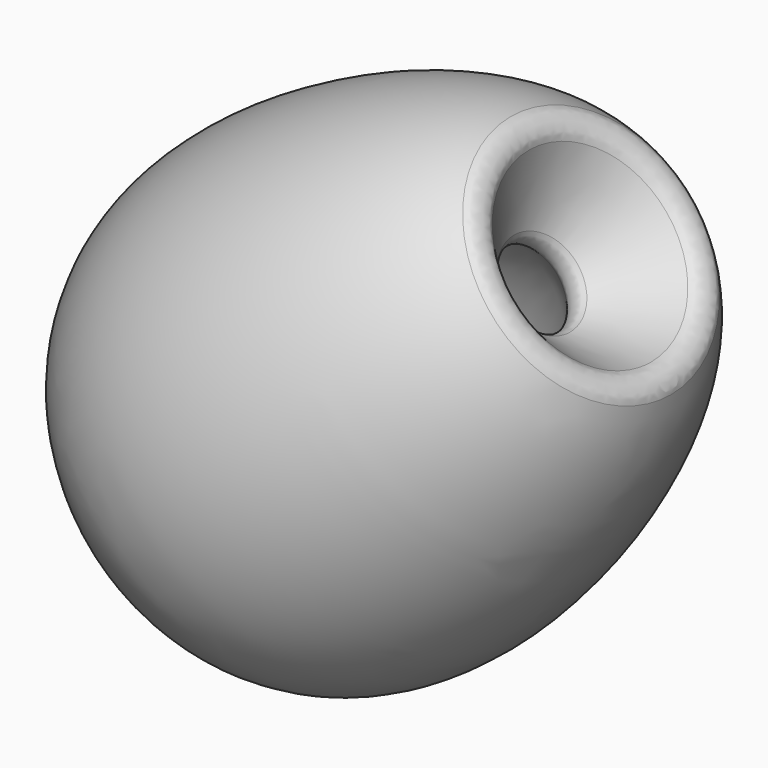
from build123d import *

# Parameters (mm, degrees)
F2_R = 12.7


# Not quite as in the source:
# - the dataset's text gives a spline's control points without its knots; the knots are read off the source's solid


with BuildPart() as f1:
    # F0 (on Front) → F1 (revolve)
    with BuildSketch(Plane.XZ):
        with BuildLine():
            add(Edge.make_bspline(
                [(-101.3375095095, -20.5878382494), (-55.6885989604, -31.3633607521), (25.6624904905, 78.1751456829), (25.6624904905, 131.8121617506)],
                knots=[0, 0, 0, 0, 198.380341768, 198.380341768, 198.380341768, 198.380341768], degree=3))
            Line((-101.3375095095, -20.5878382494), (-118.843568713, -94.7496740625))
            add(Edge.make_bspline(
                [(-118.843568713, -94.7496740625), (-116.0665941497, -95.4051848192), (-110.5257544065, -96.4677086889), (-102.3704459239, -97.3610907466), (-94.4611771904, -97.6207116792), (-86.8589683948, -97.3240119803), (-79.5982708953, -96.5506288996), (-70.3884403509, -94.9831314605), (-59.7532470515, -92.1906012776), (-48.2436048503, -87.9256433043), (-37.7728593934, -83.0146660473), (-28.1393493281, -77.6220391827), (-19.1737656331, -71.8451920299), (-10.7436627877, -65.7423860316), (-2.7492840154, -59.349854765), (4.8826869498, -52.6920953283), (14.6444972187, -43.4861585595), (26.1666233679, -31.4017634463), (39.0643071657, -16.0933493701), (51.0723883895, -0.0902528239), (62.1670566032, 16.5032811769), (72.2835752268, 33.6088961345), (79.8216178481, 48.2670302643), (85.2526772661, 60.2737062446), (89.0045449002, 69.4447684498), (92.4079357388, 78.8195768972), (95.425724145, 88.4548766457), (98.0045512843, 98.430804011), (100.0640809873, 108.856607232), (101.4793909888, 119.8740724547), (101.8624904905, 127.7282488634), (101.8624904905, 131.8121617506)],
                knots=[0, 0, 0, 0, 0.015625, 0.03125, 0.046875, 0.0625, 0.078125, 0.09375, 0.125, 0.15625, 0.1875, 0.21875, 0.25, 0.28125, 0.3125, 0.34375, 0.375, 0.4375, 0.5, 0.5625, 0.625, 0.6875, 0.75, 0.78125, 0.8125, 0.84375, 0.875, 0.90625, 0.9375, 0.96875, 1, 1, 1, 1], degree=3))
            Line((101.8624904905, 131.8121617506), (25.6624904905, 131.8121617506))
        make_face()
    revolve(axis=Axis((-88.8671576977, 0, 63.0316156894), (0.7692921059, 0, 0.6388972185)))

    # F2
    f2_edges = [f1.edges().sort_by_distance(p)[0] for p in [
        (-249.470009, 0, 62.536797),
        (-173.354659, 0, 66.127557),
        (-110.090539, 0, -57.668756),
        (-0.226063, 0, 162.984405),
        (13.765834, 0, 237.88879),
        (63.76249, 0, 131.812162),
    ]]
    fillet(f2_edges, radius=F2_R)


solid = f1.part
